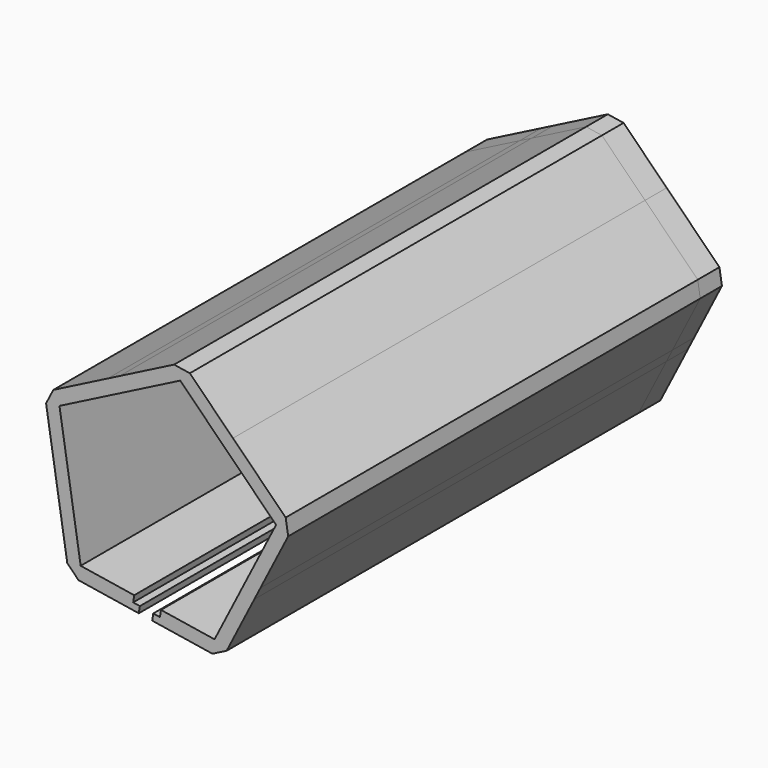
from build123d import *

# Parameters (mm, degrees)
F1_DEPTH = 101.6
F2_DEPTH = 5.08


with BuildPart() as f1:
    # F0 (on Front) → F1 (new body)
    with BuildSketch(Plane.XZ):
        Polygon((-28.6679874819, 40.9869131927), (-27.5148516125, 38.7237566213), (-4.8832858982, 50.2551153147), (-6.0364217675, 52.5182718861), (-16.220626339, 47.3291604741), (-18.4837829104, 46.1760246048), align=None)
        Polygon((-6.0364217675, 52.5182718861), (-4.8832858982, 50.2551153147), (-3.0872346739, 52.0511665389), align=None)
        Polygon((-3.0872346739, 52.0511665389), (-4.8832858982, 50.2551153147), (13.077226344, 32.2946030725), (14.8732775682, 34.0906542967), (6.7910470592, 42.1728848057), (4.994995835, 43.9689360299), align=None)
        Polygon((14.8732775682, 34.0906542967), (13.077226344, 32.2946030725), (15.3403829154, 31.1414672032), align=None)
        Polygon((15.3403829154, 31.1414672032), (13.077226344, 32.2946030725), (1.5458676506, 9.6630373581), (3.809024222, 8.5099014888), (8.9981356341, 18.6941060603), (10.1512715034, 20.9572626317), align=None)
        Polygon((-30.0235799977, 38.3264130801), (-27.5148516125, 38.7237566213), (-28.6679874819, 40.9869131927), align=None)
        Polygon((-23.5414162005, 13.6364727702), (-27.5148516125, 38.7237566213), (-30.0235799977, 38.3264130801), (-28.2355340622, 27.0371353471), (-27.838190521, 24.528406962), (-26.0501445856, 13.239129229), align=None)
        Polygon((-23.9387597417, 11.1277443851), (-23.5414162005, 13.6364727702), (-26.0501445856, 13.239129229), align=None)
        Polygon((-13.5065026601, 12.0470986054), (-23.5414162005, 13.6364727702), (-23.9387597417, 11.1277443851), (-12.6494820087, 9.3396984497), (-12.4508102381, 10.5940626422), (-13.7051744307, 10.7927344128), align=None)
        Polygon((3.809024222, 8.5099014888), (1.5458676506, 9.6630373581), (1.1485241094, 7.154308973), align=None)
        Polygon((1.5458676506, 9.6630373581), (-8.4890458899, 11.252411523), (-8.6877176605, 9.9980473304), (-9.942081853, 10.196719101), (-10.1407536236, 8.9423549084), (1.1485241094, 7.154308973), align=None)
    extrude(amount=F1_DEPTH)


with BuildPart() as f2:
    # F0 (on Front) → F2 (new body)
    with BuildSketch(Plane.XZ):
        Polygon((-4.8832858982, 50.2551153147), (-27.5148516125, 38.7237566213), (-23.5414162005, 13.6364727702), (-13.5065026601, 12.0470986054), (-8.4890458899, 11.252411523), (1.5458676506, 9.6630373581), (13.077226344, 32.2946030725), align=None)
        with BuildLine():
            add(Edge.make_bspline(
                [(-24.2410478902, 26.4475166861), (-24.1014147451, 26.5003988632), (-23.9344866256, 26.4169547892)],
                knots=[0, 0, 0, 1, 1, 1], degree=2))
            add(Edge.make_bspline(
                [(-23.9344866256, 26.4169547892), (-23.8245465392, 26.3619979088), (-23.763517385, 26.2778172496)],
                knots=[0, 0, 0, 1, 1, 1], degree=2))
            add(Edge.make_bspline(
                [(-23.763517385, 26.2778172496), (-23.7024882309, 26.1936365905), (-23.6979181512, 26.0929845147)],
                knots=[0, 0, 0, 1, 1, 1], degree=2))
            add(Edge.make_bspline(
                [(-23.6979181512, 26.0929845147), (-23.6933480715, 25.9923324389), (-23.7447541402, 25.8894956767)],
                knots=[0, 0, 0, 1, 1, 1], degree=2))
            Line((-23.7447541402, 25.8894956767), (-23.8776674766, 25.6236053355))
            Line((-23.8776674766, 25.6236053355), (-24.5884842175, 25.9789286021))
            Line((-24.5884842175, 25.9789286021), (-24.4709846317, 26.2139840586))
            add(Edge.make_bspline(
                [(-24.4709846317, 26.2139840586), (-24.3806810352, 26.394634509), (-24.2410478902, 26.4475166861)],
                knots=[0, 0, 0, 1, 1, 1], degree=2))
        make_face(mode=Mode.SUBTRACT)
        with BuildLine():
            Line((-23.5365275255, 26.9405958395), (-23.7311765646, 26.5512045201))
            add(Edge.make_bspline(
                [(-23.7311765646, 26.5512045201), (-23.6373803968, 26.5043176662), (-23.5669572, 26.517642507)],
                knots=[0, 0, 0, 1, 1, 1], degree=2))
            add(Edge.make_bspline(
                [(-23.5669572, 26.517642507), (-23.4965340031, 26.5309673477), (-23.4592504807, 26.6055522522)],
                knots=[0, 0, 0, 1, 1, 1], degree=2))
            add(Edge.make_bspline(
                [(-23.4592504807, 26.6055522522), (-23.4297141837, 26.6646389947), (-23.4356513358, 26.7120992744)],
                knots=[0, 0, 0, 1, 1, 1], degree=2))
            add(Edge.make_bspline(
                [(-23.4356513358, 26.7120992744), (-23.4415884879, 26.7595595541), (-23.4716176843, 26.7903093703)],
                knots=[0, 0, 0, 1, 1, 1], degree=2))
            Line((-23.4716176843, 26.7903093703), (-23.4092309675, 26.8586008524))
            add(Edge.make_bspline(
                [(-23.4092309675, 26.8586008524), (-23.3043703589, 26.7450438665), (-23.3911231438, 26.5714967404)],
                knots=[0, 0, 0, 1, 1, 1], degree=2))
            add(Edge.make_bspline(
                [(-23.3911231438, 26.5714967404), (-23.4516483425, 26.45041735), (-23.555446163, 26.4232062071)],
                knots=[0, 0, 0, 1, 1, 1], degree=2))
            add(Edge.make_bspline(
                [(-23.555446163, 26.4232062071), (-23.6592439835, 26.3959950642), (-23.8016333465, 26.4671726979)],
                knots=[0, 0, 0, 1, 1, 1], degree=2))
            add(Edge.make_bspline(
                [(-23.8016333465, 26.4671726979), (-23.9367579462, 26.5347188197), (-23.9772867589, 26.6340759995)],
                knots=[0, 0, 0, 1, 1, 1], degree=2))
            add(Edge.make_bspline(
                [(-23.9772867589, 26.6340759995), (-24.0178155717, 26.7334331793), (-23.9590657788, 26.8509609075)],
                knots=[0, 0, 0, 1, 1, 1], degree=2))
            add(Edge.make_bspline(
                [(-23.9590657788, 26.8509609075), (-23.8387416837, 27.0916667355), (-23.5486354645, 26.9466483593)],
                knots=[0, 0, 0, 1, 1, 1], degree=2))
            Line((-23.5486354645, 26.9466483593), (-23.5365275255, 26.9405958395))
        make_face(mode=Mode.SUBTRACT)
        with BuildLine():
            add(Edge.make_bspline(
                [(-23.2318323679, 27.4320627384), (-23.2023305644, 27.4299265975), (-23.1710113621, 27.4142707461)],
                knots=[0, 0, 0, 1, 1, 1], degree=2))
            add(Edge.make_bspline(
                [(-23.1710113621, 27.4142707461), (-23.0938434307, 27.3756960194), (-23.0810827573, 27.2964747541)],
                knots=[0, 0, 0, 1, 1, 1], degree=2))
            add(Edge.make_bspline(
                [(-23.0810827573, 27.2964747541), (-23.0683220839, 27.2172534888), (-23.1207772561, 27.1123180172)],
                knots=[0, 0, 0, 1, 1, 1], degree=2))
            add(Edge.make_bspline(
                [(-23.1207772561, 27.1123180172), (-23.1716991233, 27.0104498901), (-23.232918315, 26.9719426237)],
                knots=[0, 0, 0, 1, 1, 1], degree=2))
            add(Edge.make_bspline(
                [(-23.232918315, 26.9719426237), (-23.2941375067, 26.9334353572), (-23.3736443155, 26.9523959378)],
                knots=[0, 0, 0, 1, 1, 1], degree=2))
            Line((-23.3736443155, 26.9523959378), (-23.3491958849, 27.0404591395))
            add(Edge.make_bspline(
                [(-23.3491958849, 27.0404591395), (-23.299474007, 27.0301322889), (-23.2608943902, 27.0562475224)],
                knots=[0, 0, 0, 1, 1, 1], degree=2))
            add(Edge.make_bspline(
                [(-23.2608943902, 27.0562475224), (-23.2223147734, 27.082362756), (-23.1900346674, 27.1469384309)],
                knots=[0, 0, 0, 1, 1, 1], degree=2))
            add(Edge.make_bspline(
                [(-23.1900346674, 27.1469384309), (-23.155494954, 27.216034403), (-23.1606244849, 27.2586518163)],
                knots=[0, 0, 0, 1, 1, 1], degree=2))
            add(Edge.make_bspline(
                [(-23.1606244849, 27.2586518163), (-23.1657540158, 27.3012692297), (-23.208212522, 27.3224933994)],
                knots=[0, 0, 0, 1, 1, 1], degree=2))
            add(Edge.make_bspline(
                [(-23.208212522, 27.3224933994), (-23.2405003595, 27.3386334523), (-23.2717765443, 27.3265230972)],
                knots=[0, 0, 0, 1, 1, 1], degree=2))
            add(Edge.make_bspline(
                [(-23.2717765443, 27.3265230972), (-23.3030527291, 27.3144127421), (-23.3408235843, 27.2715490723)],
                knots=[0, 0, 0, 1, 1, 1], degree=2))
            Line((-23.3408235843, 27.2715490723), (-23.390458345, 27.215043308))
            add(Edge.make_bspline(
                [(-23.390458345, 27.215043308), (-23.4497778719, 27.1468328354), (-23.4857344981, 27.1235429035)],
                knots=[0, 0, 0, 1, 1, 1], degree=2))
            add(Edge.make_bspline(
                [(-23.4857344981, 27.1235429035), (-23.5216911243, 27.1002529717), (-23.5587795451, 27.0954871912)],
                knots=[0, 0, 0, 1, 1, 1], degree=2))
            add(Edge.make_bspline(
                [(-23.5587795451, 27.0954871912), (-23.5958679659, 27.0907214106), (-23.6362277627, 27.1108964769)],
                knots=[0, 0, 0, 1, 1, 1], degree=2))
            add(Edge.make_bspline(
                [(-23.6362277627, 27.1108964769), (-23.7108126671, 27.1481799993), (-23.7232902131, 27.2209036756)],
                knots=[0, 0, 0, 1, 1, 1], degree=2))
            add(Edge.make_bspline(
                [(-23.7232902131, 27.2209036756), (-23.7357677591, 27.2936273518), (-23.6848458919, 27.3954954789)],
                knots=[0, 0, 0, 1, 1, 1], degree=2))
            add(Edge.make_bspline(
                [(-23.6848458919, 27.3954954789), (-23.6396537435, 27.4859014237), (-23.5813402059, 27.5232380338)],
                knots=[0, 0, 0, 1, 1, 1], degree=2))
            add(Edge.make_bspline(
                [(-23.5813402059, 27.5232380338), (-23.5230266683, 27.5605746439), (-23.4457796989, 27.5395152379)],
                knots=[0, 0, 0, 1, 1, 1], degree=2))
            Line((-23.4457796989, 27.5395152379), (-23.4766048034, 27.4528235928))
            add(Edge.make_bspline(
                [(-23.4766048034, 27.4528235928), (-23.5167215329, 27.4633935106), (-23.5525974396, 27.4400632286)],
                knots=[0, 0, 0, 1, 1, 1], degree=2))
            add(Edge.make_bspline(
                [(-23.5525974396, 27.4400632286), (-23.5884733462, 27.4167329467), (-23.6162342374, 27.3611978663)],
                knots=[0, 0, 0, 1, 1, 1], degree=2))
            add(Edge.make_bspline(
                [(-23.6162342374, 27.3611978663), (-23.6469810383, 27.299689536), (-23.6429819103, 27.2610674429)],
                knots=[0, 0, 0, 1, 1, 1], degree=2))
            add(Edge.make_bspline(
                [(-23.6429819103, 27.2610674429), (-23.6389827823, 27.2224453499), (-23.6012060125, 27.2035614879)],
                knots=[0, 0, 0, 1, 1, 1], degree=2))
            add(Edge.make_bspline(
                [(-23.6012060125, 27.2035614879), (-23.5779587695, 27.1919406497), (-23.5568116857, 27.196503114)],
                knots=[0, 0, 0, 1, 1, 1], degree=2))
            add(Edge.make_bspline(
                [(-23.5568116857, 27.196503114), (-23.5356646018, 27.2010655782), (-23.5131466765, 27.2194709213)],
                knots=[0, 0, 0, 1, 1, 1], degree=2))
            add(Edge.make_bspline(
                [(-23.5131466765, 27.2194709213), (-23.4906287512, 27.2378762643), (-23.4339727196, 27.3047950301)],
                knots=[0, 0, 0, 1, 1, 1], degree=2))
            add(Edge.make_bspline(
                [(-23.4339727196, 27.3047950301), (-23.379657073, 27.3678392168), (-23.3484223981, 27.3919762115)],
                knots=[0, 0, 0, 1, 1, 1], degree=2))
            add(Edge.make_bspline(
                [(-23.3484223981, 27.3919762115), (-23.3171877231, 27.4161132062), (-23.2892609472, 27.4251560428)],
                knots=[0, 0, 0, 1, 1, 1], degree=2))
            add(Edge.make_bspline(
                [(-23.2892609472, 27.4251560428), (-23.2613341713, 27.4341988794), (-23.2318323679, 27.4320627384)],
                knots=[0, 0, 0, 1, 1, 1], degree=2))
        make_face(mode=Mode.SUBTRACT)
        Polygon((-22.9216114376, 27.5361753853), (-22.9670456868, 27.4452851229), (-23.5128715784, 27.7181327188), (-23.4674373292, 27.8090229811), align=None, mode=Mode.SUBTRACT)
        Polygon((-23.5835121048, 27.8670464716), (-23.6289463539, 27.7761562093), (-23.7158006366, 27.8195729518), (-23.6703663874, 27.9104632142), align=None, mode=Mode.SUBTRACT)
        with BuildLine():
            add(Edge.make_bspline(
                [(-22.6500587957, 28.1185653779), (-22.4200079541, 28.0035675003), (-22.534198829, 27.7751310506)],
                knots=[0, 0, 0, 1, 1, 1], degree=2))
            add(Edge.make_bspline(
                [(-22.534198829, 27.7751310506), (-22.5789067758, 27.6856937409), (-22.6404087663, 27.650253645)],
                knots=[0, 0, 0, 1, 1, 1], degree=2))
            add(Edge.make_bspline(
                [(-22.6404087663, 27.650253645), (-22.7019107568, 27.6148135492), (-22.7740722566, 27.6319183716)],
                knots=[0, 0, 0, 1, 1, 1], degree=2))
            Line((-22.7740722566, 27.6319183716), (-22.7414724808, 27.7298296729))
            add(Edge.make_bspline(
                [(-22.7414724808, 27.7298296729), (-22.6991764961, 27.7199864054), (-22.663219638, 27.7408548654)],
                knots=[0, 0, 0, 1, 1, 1], degree=2))
            add(Edge.make_bspline(
                [(-22.663219638, 27.7408548654), (-22.6272627798, 27.7617233254), (-22.6020842971, 27.8120923518)],
                knots=[0, 0, 0, 1, 1, 1], degree=2))
            add(Edge.make_bspline(
                [(-22.6020842971, 27.8120923518), (-22.5342153743, 27.9478627082), (-22.6930715344, 28.0272717689)],
                knots=[0, 0, 0, 1, 1, 1], degree=2))
            Line((-22.6930715344, 28.0272717689), (-22.7808944522, 28.071172713))
            Line((-22.7808944522, 28.071172713), (-22.7813786538, 28.0702040779))
            add(Edge.make_bspline(
                [(-22.7813786538, 28.0702040779), (-22.7418229604, 28.0181462218), (-22.7377816073, 27.9600312844)],
                knots=[0, 0, 0, 1, 1, 1], degree=2))
            add(Edge.make_bspline(
                [(-22.7377816073, 27.9600312844), (-22.7337402543, 27.9019163469), (-22.7637607529, 27.8418609693)],
                knots=[0, 0, 0, 1, 1, 1], degree=2))
            add(Edge.make_bspline(
                [(-22.7637607529, 27.8418609693), (-22.8139563177, 27.7414457949), (-22.9041144597, 27.7275944116)],
                knots=[0, 0, 0, 1, 1, 1], degree=2))
            add(Edge.make_bspline(
                [(-22.9041144597, 27.7275944116), (-22.9942726018, 27.7137430282), (-23.1369848432, 27.7850820625)],
                knots=[0, 0, 0, 1, 1, 1], degree=2))
            add(Edge.make_bspline(
                [(-23.1369848432, 27.7850820625), (-23.2817957941, 27.8574702001), (-23.3253097242, 27.9425807679)],
                knots=[0, 0, 0, 1, 1, 1], degree=2))
            add(Edge.make_bspline(
                [(-23.3253097242, 27.9425807679), (-23.3688236543, 28.0276913357), (-23.3170947844, 28.1311738546)],
                knots=[0, 0, 0, 1, 1, 1], degree=2))
            add(Edge.make_bspline(
                [(-23.3170947844, 28.1311738546), (-23.2881233893, 28.1891305228), (-23.2403424927, 28.2185156247)],
                knots=[0, 0, 0, 1, 1, 1], degree=2))
            add(Edge.make_bspline(
                [(-23.2403424927, 28.2185156247), (-23.192561596, 28.2479007267), (-23.1320246842, 28.2466957893)],
                knots=[0, 0, 0, 1, 1, 1], degree=2))
            Line((-23.1320246842, 28.2466957893), (-23.1315404826, 28.2476644244))
            add(Edge.make_bspline(
                [(-23.1315404826, 28.2476644244), (-23.1467157662, 28.2552502494), (-23.1829994651, 28.2759100004)],
                knots=[0, 0, 0, 1, 1, 1], degree=2))
            add(Edge.make_bspline(
                [(-23.1829994651, 28.2759100004), (-23.219283164, 28.2965697514), (-23.2217857227, 28.3004438667)],
                knots=[0, 0, 0, 1, 1, 1], degree=2))
            Line((-23.2217857227, 28.3004438667), (-23.1786917812, 28.3866523926))
            add(Edge.make_bspline(
                [(-23.1786917812, 28.3866523926), (-23.1531033028, 28.3700274036), (-23.0672176552, 28.3270948626)],
                knots=[0, 0, 0, 1, 1, 1], degree=2))
            Line((-23.0672176552, 28.3270948626), (-22.6500587957, 28.1185653779))
        make_face(mode=Mode.SUBTRACT)
        with BuildLine():
            Line((-22.3458957473, 28.6878825462), (-22.3915720973, 28.5965079663))
            Line((-22.3915720973, 28.5965079663), (-22.7376977145, 28.7695293343))
            add(Edge.make_bspline(
                [(-22.7376977145, 28.7695293343), (-22.791618403, 28.7964832228), (-22.8266898003, 28.800798155)],
                knots=[0, 0, 0, 1, 1, 1], degree=2))
            add(Edge.make_bspline(
                [(-22.8266898003, 28.800798155), (-22.8617611977, 28.8051130871), (-22.88645861, 28.7884025656)],
                knots=[0, 0, 0, 1, 1, 1], degree=2))
            add(Edge.make_bspline(
                [(-22.88645861, 28.7884025656), (-22.9111560223, 28.7716920441), (-22.933590696, 28.7268119501)],
                knots=[0, 0, 0, 1, 1, 1], degree=2))
            add(Edge.make_bspline(
                [(-22.933590696, 28.7268119501), (-22.9663550036, 28.6612676402), (-22.9403991217, 28.6009754771)],
                knots=[0, 0, 0, 1, 1, 1], degree=2))
            add(Edge.make_bspline(
                [(-22.9403991217, 28.6009754771), (-22.9144432398, 28.5406833141), (-22.8346922814, 28.5008173832)],
                knots=[0, 0, 0, 1, 1, 1], degree=2))
            Line((-22.8346922814, 28.5008173832), (-22.5184329138, 28.3427255641))
            Line((-22.5184329138, 28.3427255641), (-22.5637864627, 28.251996741))
            Line((-22.5637864627, 28.251996741), (-22.9930532613, 28.4665787455))
            add(Edge.make_bspline(
                [(-22.9930532613, 28.4665787455), (-23.0884638209, 28.5142726021), (-23.1111456594, 28.5217769922)],
                knots=[0, 0, 0, 1, 1, 1], degree=2))
            Line((-23.1111456594, 28.5217769922), (-23.0682938187, 28.6075012006))
            add(Edge.make_bspline(
                [(-23.0682938187, 28.6075012006), (-23.0656301301, 28.6067750142), (-23.0542083753, 28.6017717331)],
                knots=[0, 0, 0, 1, 1, 1], degree=2))
            add(Edge.make_bspline(
                [(-23.0542083753, 28.6017717331), (-23.0427866204, 28.5967684519), (-23.0280553816, 28.5903126047)],
                knots=[0, 0, 0, 1, 1, 1], degree=2))
            add(Edge.make_bspline(
                [(-23.0280553816, 28.5903126047), (-23.0133241427, 28.5838567575), (-22.9729644619, 28.5648924271)],
                knots=[0, 0, 0, 1, 1, 1], degree=2))
            Line((-22.9729644619, 28.5648924271), (-22.9721574593, 28.566506819))
            add(Edge.make_bspline(
                [(-22.9721574593, 28.566506819), (-23.0130860236, 28.6259096749), (-23.0159968578, 28.6788185561)],
                knots=[0, 0, 0, 1, 1, 1], degree=2))
            add(Edge.make_bspline(
                [(-23.0159968578, 28.6788185561), (-23.0189076919, 28.7317274374), (-22.9884029918, 28.7927514501)],
                knots=[0, 0, 0, 1, 1, 1], degree=2))
            add(Edge.make_bspline(
                [(-22.9884029918, 28.7927514501), (-22.9435336445, 28.8825116382), (-22.8780750409, 28.9018493252)],
                knots=[0, 0, 0, 1, 1, 1], degree=2))
            add(Edge.make_bspline(
                [(-22.8780750409, 28.9018493252), (-22.8126164373, 28.9211870122), (-22.7096182359, 28.8697002431)],
                knots=[0, 0, 0, 1, 1, 1], degree=2))
            Line((-22.7096182359, 28.8697002431), (-22.3458957473, 28.6878825462))
        make_face(mode=Mode.SUBTRACT)
        with BuildLine():
            Line((-22.3018941717, 29.4104539632), (-22.4965432108, 29.0210626438))
            add(Edge.make_bspline(
                [(-22.4965432108, 29.0210626438), (-22.4027470431, 28.9741757899), (-22.3323238463, 28.9875006307)],
                knots=[0, 0, 0, 1, 1, 1], degree=2))
            add(Edge.make_bspline(
                [(-22.3323238463, 28.9875006307), (-22.2619006494, 29.0008254714), (-22.224617127, 29.0754103759)],
                knots=[0, 0, 0, 1, 1, 1], degree=2))
            add(Edge.make_bspline(
                [(-22.224617127, 29.0754103759), (-22.19508083, 29.1344971184), (-22.2010179821, 29.1819573981)],
                knots=[0, 0, 0, 1, 1, 1], degree=2))
            add(Edge.make_bspline(
                [(-22.2010179821, 29.1819573981), (-22.2069551342, 29.2294176778), (-22.2369843306, 29.260167494)],
                knots=[0, 0, 0, 1, 1, 1], degree=2))
            Line((-22.2369843306, 29.260167494), (-22.1745976138, 29.3284589761))
            add(Edge.make_bspline(
                [(-22.1745976138, 29.3284589761), (-22.0697370052, 29.2149019902), (-22.15648979, 29.0413548641)],
                knots=[0, 0, 0, 1, 1, 1], degree=2))
            add(Edge.make_bspline(
                [(-22.15648979, 29.0413548641), (-22.2170149888, 28.9202754737), (-22.3208128093, 28.8930643308)],
                knots=[0, 0, 0, 1, 1, 1], degree=2))
            add(Edge.make_bspline(
                [(-22.3208128093, 28.8930643308), (-22.4246106298, 28.8658531879), (-22.5669999928, 28.9370308216)],
                knots=[0, 0, 0, 1, 1, 1], degree=2))
            add(Edge.make_bspline(
                [(-22.5669999928, 28.9370308216), (-22.7021245924, 29.0045769434), (-22.7426534052, 29.1039341232)],
                knots=[0, 0, 0, 1, 1, 1], degree=2))
            add(Edge.make_bspline(
                [(-22.7426534052, 29.1039341232), (-22.783182218, 29.203291303), (-22.7244324251, 29.3208190312)],
                knots=[0, 0, 0, 1, 1, 1], degree=2))
            add(Edge.make_bspline(
                [(-22.7244324251, 29.3208190312), (-22.60410833, 29.5615248592), (-22.3140021108, 29.416506483)],
                knots=[0, 0, 0, 1, 1, 1], degree=2))
            Line((-22.3140021108, 29.416506483), (-22.3018941717, 29.4104539632))
        make_face(mode=Mode.SUBTRACT)
        with BuildLine():
            Line((-21.9049705291, 29.7895330443), (-21.9059389322, 29.7875957741))
            add(Edge.make_bspline(
                [(-21.9059389322, 29.7875957741), (-21.866141138, 29.7360222356), (-21.8641585309, 29.6830729075)],
                knots=[0, 0, 0, 1, 1, 1], degree=2))
            add(Edge.make_bspline(
                [(-21.8641585309, 29.6830729075), (-21.8621759237, 29.6301235795), (-21.8929227247, 29.5686152492)],
                knots=[0, 0, 0, 1, 1, 1], degree=2))
            add(Edge.make_bspline(
                [(-21.8929227247, 29.5686152492), (-21.9446515945, 29.4651327302), (-22.0386437336, 29.4512809797)],
                knots=[0, 0, 0, 1, 1, 1], degree=2))
            add(Edge.make_bspline(
                [(-22.0386437336, 29.4512809797), (-22.1326358728, 29.4374292291), (-22.2738951615, 29.5080419609)],
                knots=[0, 0, 0, 1, 1, 1], degree=2))
            add(Edge.make_bspline(
                [(-22.2738951615, 29.5080419609), (-22.5594810835, 29.6508007296), (-22.4590899539, 29.8516310784)],
                knots=[0, 0, 0, 1, 1, 1], degree=2))
            add(Edge.make_bspline(
                [(-22.4590899539, 29.8516310784), (-22.4281010521, 29.9136237263), (-22.3847595785, 29.9436137709)],
                knots=[0, 0, 0, 1, 1, 1], degree=2))
            add(Edge.make_bspline(
                [(-22.3847595785, 29.9436137709), (-22.3414181049, 29.9736038156), (-22.2791863328, 29.9741747867)],
                knots=[0, 0, 0, 1, 1, 1], degree=2))
            Line((-22.2791863328, 29.9741747867), (-22.2787021313, 29.9751434218))
            Line((-22.2787021313, 29.9751434218), (-22.3402103456, 30.0046794868))
            Line((-22.3402103456, 30.0046794868), (-22.5668709643, 30.1179826588))
            Line((-22.5668709643, 30.1179826588), (-22.5215174154, 30.208711482))
            Line((-22.5215174154, 30.208711482), (-21.8852855789, 29.8906717378))
            add(Edge.make_bspline(
                [(-21.8852855789, 29.8906717378), (-21.8000456882, 29.8480619979), (-21.7712291605, 29.8374909976)],
                knots=[0, 0, 0, 1, 1, 1], degree=2))
            Line((-21.7712291605, 29.8374909976), (-21.814645903, 29.750636715))
            add(Edge.make_bspline(
                [(-21.814645903, 29.750636715), (-21.8234441648, 29.7532187755), (-21.8536330802, 29.7660900426)],
                knots=[0, 0, 0, 1, 1, 1], degree=2))
            add(Edge.make_bspline(
                [(-21.8536330802, 29.7660900426), (-21.8838219955, 29.7789613096), (-21.9049705291, 29.7895330443)],
                knots=[0, 0, 0, 1, 1, 1], degree=2))
        make_face(mode=Mode.SUBTRACT)
        with BuildLine():
            add(Edge.make_bspline(
                [(-21.8395776893, 30.9167748155), (-21.7455855502, 30.9306265661), (-21.6043262614, 30.8600138342)],
                knots=[0, 0, 0, 1, 1, 1], degree=2))
            add(Edge.make_bspline(
                [(-21.6043262614, 30.8600138342), (-21.3187403394, 30.7172550655), (-21.419131469, 30.5164247168)],
                knots=[0, 0, 0, 1, 1, 1], degree=2))
            add(Edge.make_bspline(
                [(-21.419131469, 30.5164247168), (-21.4501203708, 30.4544320689), (-21.493219705, 30.4245227631)],
                knots=[0, 0, 0, 1, 1, 1], degree=2))
            add(Edge.make_bspline(
                [(-21.493219705, 30.4245227631), (-21.5363190391, 30.3946134574), (-21.5990350901, 30.3938810085)],
                knots=[0, 0, 0, 1, 1, 1], degree=2))
            Line((-21.5990350901, 30.3938810085), (-21.5995192917, 30.3929123734))
            add(Edge.make_bspline(
                [(-21.5995192917, 30.3929123734), (-21.5838596905, 30.3850844477), (-21.5528227652, 30.3670474553)],
                knots=[0, 0, 0, 1, 1, 1], degree=2))
            add(Edge.make_bspline(
                [(-21.5528227652, 30.3670474553), (-21.5217858399, 30.3490104628), (-21.5173461269, 30.3453786803)],
                knots=[0, 0, 0, 1, 1, 1], degree=2))
            Line((-21.5173461269, 30.3453786803), (-21.5611663708, 30.2577172017))
            add(Edge.make_bspline(
                [(-21.5611663708, 30.2577172017), (-21.5869969886, 30.2742614518), (-21.6722368794, 30.3168711917)],
                knots=[0, 0, 0, 1, 1, 1], degree=2))
            Line((-21.6722368794, 30.3168711917), (-22.3084687159, 30.634910936))
            Line((-22.3084687159, 30.634910936), (-22.2630344667, 30.7258011983))
            Line((-22.2630344667, 30.7258011983), (-22.0496118613, 30.619115448))
            add(Edge.make_bspline(
                [(-22.0496118613, 30.619115448), (-22.0168397063, 30.6027332942), (-21.9734930333, 30.578442012)],
                knots=[0, 0, 0, 1, 1, 1], degree=2))
            Line((-21.9734930333, 30.578442012), (-21.9724439299, 30.5805407214))
            add(Edge.make_bspline(
                [(-21.9724439299, 30.5805407214), (-22.0123224244, 30.6319528207), (-22.0141839618, 30.6849425182)],
                knots=[0, 0, 0, 1, 1, 1], degree=2))
            add(Edge.make_bspline(
                [(-22.0141839618, 30.6849425182), (-22.0160454992, 30.7379322157), (-21.9852986983, 30.799440546)],
                knots=[0, 0, 0, 1, 1, 1], degree=2))
            add(Edge.make_bspline(
                [(-21.9852986983, 30.799440546), (-21.9335698284, 30.9029230649), (-21.8395776893, 30.9167748155)],
                knots=[0, 0, 0, 1, 1, 1], degree=2))
        make_face(mode=Mode.SUBTRACT)
        with BuildLine():
            add(Edge.make_bspline(
                [(-21.0253913312, 30.8457422463), (-21.0222793649, 30.7996942212), (-21.0447140385, 30.7548141272)],
                knots=[0, 0, 0, 1, 1, 1], degree=2))
            add(Edge.make_bspline(
                [(-21.0447140385, 30.7548141272), (-21.0633557997, 30.717521675), (-21.0815146737, 30.6949195316)],
                knots=[0, 0, 0, 1, 1, 1], degree=2))
            Line((-21.0815146737, 30.6949195316), (-21.1496420107, 30.7289750434))
            add(Edge.make_bspline(
                [(-21.1496420107, 30.7289750434), (-21.1369713346, 30.7466530017), (-21.1253504964, 30.7699002446)],
                knots=[0, 0, 0, 1, 1, 1], degree=2))
            add(Edge.make_bspline(
                [(-21.1253504964, 30.7699002446), (-21.0829828573, 30.8546558178), (-21.1829196287, 30.9663568136)],
                knots=[0, 0, 0, 1, 1, 1], degree=2))
            Line((-21.1829196287, 30.9663568136), (-21.2004368049, 30.9858076263))
            Line((-21.2004368049, 30.9858076263), (-21.8518180246, 31.0410355072))
            Line((-21.8518180246, 31.0410355072), (-21.8033978656, 31.1378990195))
            Line((-21.8033978656, 31.1378990195), (-21.4443708754, 31.1020956257))
            add(Edge.make_bspline(
                [(-21.4443708754, 31.1020956257), (-21.435976347, 31.1011278411), (-21.4243531507, 31.099756787)],
                knots=[0, 0, 0, 1, 1, 1], degree=2))
            add(Edge.make_bspline(
                [(-21.4243531507, 31.099756787), (-21.4127299545, 31.098385733), (-21.3471475751, 31.0895132847)],
                knots=[0, 0, 0, 1, 1, 1], degree=2))
            add(Edge.make_bspline(
                [(-21.3471475751, 31.0895132847), (-21.2815651958, 31.0806408365), (-21.274381326, 31.0788657785)],
                knots=[0, 0, 0, 1, 1, 1], degree=2))
            Line((-21.274381326, 31.0788657785), (-21.355993068, 31.1638516235))
            Line((-21.355993068, 31.1638516235), (-21.6437727415, 31.4572257316))
            Line((-21.6437727415, 31.4572257316), (-21.5958367841, 31.5531206087))
            Line((-21.5958367841, 31.5531206087), (-21.1549212369, 31.0704020696))
            add(Edge.make_bspline(
                [(-21.1549212369, 31.0704020696), (-21.0845296924, 30.992840997), (-21.0565164949, 30.9423156342)],
                knots=[0, 0, 0, 1, 1, 1], degree=2))
            add(Edge.make_bspline(
                [(-21.0565164949, 30.9423156342), (-21.0285032975, 30.8917902714), (-21.0253913312, 30.8457422463)],
                knots=[0, 0, 0, 1, 1, 1], degree=2))
        make_face(mode=Mode.SUBTRACT)
        with BuildLine():
            add(Edge.make_bspline(
                [(-20.7628104206, 31.9777247755), (-20.7314845113, 31.8920480302), (-20.780146771, 31.7947002003)],
                knots=[0, 0, 0, 1, 1, 1], degree=2))
            add(Edge.make_bspline(
                [(-20.780146771, 31.7947002003), (-20.8704503675, 31.61404975), (-21.0741018624, 31.6736791664)],
                knots=[0, 0, 0, 1, 1, 1], degree=2))
            Line((-21.0741018624, 31.6736791664), (-21.0426325088, 31.7757875774))
            add(Edge.make_bspline(
                [(-21.0426325088, 31.7757875774), (-20.9794301688, 31.7556954149), (-20.9308004117, 31.7710360614)],
                knots=[0, 0, 0, 1, 1, 1], degree=2))
            add(Edge.make_bspline(
                [(-20.9308004117, 31.7710360614), (-20.8821706547, 31.7863767078), (-20.858202676, 31.8343241464)],
                knots=[0, 0, 0, 1, 1, 1], degree=2))
            add(Edge.make_bspline(
                [(-20.858202676, 31.8343241464), (-20.8319750899, 31.8867918822), (-20.8529254485, 31.935098239)],
                knots=[0, 0, 0, 1, 1, 1], degree=2))
            add(Edge.make_bspline(
                [(-20.8529254485, 31.935098239), (-20.8738758072, 31.9834045958), (-20.9434560968, 32.01818641)],
                knots=[0, 0, 0, 1, 1, 1], degree=2))
            Line((-20.9434560968, 32.01818641), (-21.3657810103, 32.2292983032))
            Line((-21.3657810103, 32.2292983032), (-21.4341341347, 32.0925593117))
            Line((-21.4341341347, 32.0925593117), (-21.5127550189, 32.1318603407))
            Line((-21.5127550189, 32.1318603407), (-21.396465937, 32.3644942094))
            Line((-21.396465937, 32.3644942094), (-20.8976188489, 32.1151303906))
            add(Edge.make_bspline(
                [(-20.8976188489, 32.1151303906), (-20.7941363299, 32.0634015208), (-20.7628104206, 31.9777247755)],
                knots=[0, 0, 0, 1, 1, 1], degree=2))
        make_face(mode=Mode.SUBTRACT)
        with BuildLine():
            Line((-20.6368056047, 32.7414287109), (-20.8314546438, 32.3520373916))
            add(Edge.make_bspline(
                [(-20.8314546438, 32.3520373916), (-20.7376584761, 32.3051505377), (-20.6672352792, 32.3184753784)],
                knots=[0, 0, 0, 1, 1, 1], degree=2))
            add(Edge.make_bspline(
                [(-20.6672352792, 32.3184753784), (-20.5968120824, 32.3318002192), (-20.55952856, 32.4063851237)],
                knots=[0, 0, 0, 1, 1, 1], degree=2))
            add(Edge.make_bspline(
                [(-20.55952856, 32.4063851237), (-20.529992263, 32.4654718661), (-20.5359294151, 32.5129321459)],
                knots=[0, 0, 0, 1, 1, 1], degree=2))
            add(Edge.make_bspline(
                [(-20.5359294151, 32.5129321459), (-20.5418665671, 32.5603924256), (-20.5718957636, 32.5911422418)],
                knots=[0, 0, 0, 1, 1, 1], degree=2))
            Line((-20.5718957636, 32.5911422418), (-20.5095090467, 32.6594337239))
            add(Edge.make_bspline(
                [(-20.5095090467, 32.6594337239), (-20.4046484382, 32.545876738), (-20.491401223, 32.3723296118)],
                knots=[0, 0, 0, 1, 1, 1], degree=2))
            add(Edge.make_bspline(
                [(-20.491401223, 32.3723296118), (-20.5519264217, 32.2512502215), (-20.6557242422, 32.2240390786)],
                knots=[0, 0, 0, 1, 1, 1], degree=2))
            add(Edge.make_bspline(
                [(-20.6557242422, 32.2240390786), (-20.7595220627, 32.1968279357), (-20.9019114258, 32.2680055694)],
                knots=[0, 0, 0, 1, 1, 1], degree=2))
            add(Edge.make_bspline(
                [(-20.9019114258, 32.2680055694), (-21.0370360254, 32.3355516912), (-21.0775648382, 32.434908871)],
                knots=[0, 0, 0, 1, 1, 1], degree=2))
            add(Edge.make_bspline(
                [(-21.0775648382, 32.434908871), (-21.1180936509, 32.5342660507), (-21.059343858, 32.651793779)],
                knots=[0, 0, 0, 1, 1, 1], degree=2))
            add(Edge.make_bspline(
                [(-21.059343858, 32.651793779), (-20.939019763, 32.892499607), (-20.6489135437, 32.7474812308)],
                knots=[0, 0, 0, 1, 1, 1], degree=2))
            Line((-20.6489135437, 32.7474812308), (-20.6368056047, 32.7414287109))
        make_face(mode=Mode.SUBTRACT)
        with BuildLine():
            Line((-20.6956095176, 33.1889110776), (-20.7488716925, 33.0823612141))
            Line((-20.7488716925, 33.0823612141), (-20.2690744284, 32.8425200266))
            Line((-20.2690744284, 32.8425200266), (-20.3144279773, 32.7517912035))
            Line((-20.3144279773, 32.7517912035), (-20.7942252414, 32.9916323909))
            Line((-20.7942252414, 32.9916323909), (-20.8325578673, 32.9149487771))
            Line((-20.8325578673, 32.9149487771), (-20.8985864948, 32.9479551854))
            Line((-20.8985864948, 32.9479551854), (-20.860253869, 33.0246387993))
            Line((-20.860253869, 33.0246387993), (-20.9219236384, 33.0554663005))
            add(Edge.make_bspline(
                [(-20.9219236384, 33.0554663005), (-20.9965085429, 33.0927498229), (-21.0128985441, 33.1419041317)],
                knots=[0, 0, 0, 1, 1, 1], degree=2))
            add(Edge.make_bspline(
                [(-21.0128985441, 33.1419041317), (-21.0292885453, 33.1910584405), (-20.9954751343, 33.2587014599)],
                knots=[0, 0, 0, 1, 1, 1], degree=2))
            add(Edge.make_bspline(
                [(-20.9954751343, 33.2587014599), (-20.9765912723, 33.2964782297), (-20.9574638791, 33.3198069074)],
                knots=[0, 0, 0, 1, 1, 1], degree=2))
            Line((-20.9574638791, 33.3198069074), (-20.8883679071, 33.285267194))
            add(Edge.make_bspline(
                [(-20.8883679071, 33.285267194), (-20.9037826241, 33.2645217752), (-20.912578953, 33.2469249038)],
                knots=[0, 0, 0, 1, 1, 1], degree=2))
            add(Edge.make_bspline(
                [(-20.912578953, 33.2469249038), (-20.9300102102, 33.2120540394), (-20.9201605449, 33.1875577592)],
                knots=[0, 0, 0, 1, 1, 1], degree=2))
            add(Edge.make_bspline(
                [(-20.9201605449, 33.1875577592), (-20.9103108796, 33.1630614791), (-20.8638163938, 33.1398198028)],
                knots=[0, 0, 0, 1, 1, 1], degree=2))
            Line((-20.8638163938, 33.1398198028), (-20.8149003201, 33.1153676225))
            Line((-20.8149003201, 33.1153676225), (-20.7616381452, 33.221917486))
            Line((-20.7616381452, 33.221917486), (-20.6956095176, 33.1889110776))
        make_face(mode=Mode.SUBTRACT)
        with BuildLine():
            Line((-20.5521244465, 33.4759499523), (-20.6053866214, 33.3694000888))
            Line((-20.6053866214, 33.3694000888), (-20.1255893573, 33.1295589013))
            Line((-20.1255893573, 33.1295589013), (-20.1709429062, 33.0388300782))
            Line((-20.1709429062, 33.0388300782), (-20.6507401703, 33.2786712656))
            Line((-20.6507401703, 33.2786712656), (-20.6890727962, 33.2019876518))
            Line((-20.6890727962, 33.2019876518), (-20.7551014237, 33.2349940601))
            Line((-20.7551014237, 33.2349940601), (-20.7167687979, 33.311677674))
            Line((-20.7167687979, 33.311677674), (-20.7784385673, 33.3425051752))
            add(Edge.make_bspline(
                [(-20.7784385673, 33.3425051752), (-20.8530234718, 33.3797886976), (-20.869413473, 33.4289430064)],
                knots=[0, 0, 0, 1, 1, 1], degree=2))
            add(Edge.make_bspline(
                [(-20.869413473, 33.4289430064), (-20.8858034742, 33.4780973152), (-20.8519900632, 33.5457403346)],
                knots=[0, 0, 0, 1, 1, 1], degree=2))
            add(Edge.make_bspline(
                [(-20.8519900632, 33.5457403346), (-20.8331062012, 33.5835171044), (-20.813978808, 33.6068457821)],
                knots=[0, 0, 0, 1, 1, 1], degree=2))
            Line((-20.813978808, 33.6068457821), (-20.744882836, 33.5723060687))
            add(Edge.make_bspline(
                [(-20.744882836, 33.5723060687), (-20.760297553, 33.5515606499), (-20.7690938819, 33.5339637785)],
                knots=[0, 0, 0, 1, 1, 1], degree=2))
            add(Edge.make_bspline(
                [(-20.7690938819, 33.5339637785), (-20.7865251391, 33.4990929141), (-20.7766754738, 33.4745966339)],
                knots=[0, 0, 0, 1, 1, 1], degree=2))
            add(Edge.make_bspline(
                [(-20.7766754738, 33.4745966339), (-20.7668258085, 33.4501003538), (-20.7203313226, 33.4268586775)],
                knots=[0, 0, 0, 1, 1, 1], degree=2))
            Line((-20.7203313226, 33.4268586775), (-20.6714152489, 33.4024064972))
            Line((-20.6714152489, 33.4024064972), (-20.6181530741, 33.5089563607))
            Line((-20.6181530741, 33.5089563607), (-20.5521244465, 33.4759499523))
        make_face(mode=Mode.SUBTRACT)
        with BuildLine():
            Line((-20.0626232195, 33.8900685273), (-20.2572722586, 33.500677208))
            add(Edge.make_bspline(
                [(-20.2572722586, 33.500677208), (-20.1634760908, 33.453790354), (-20.093052894, 33.4671151948)],
                knots=[0, 0, 0, 1, 1, 1], degree=2))
            add(Edge.make_bspline(
                [(-20.093052894, 33.4671151948), (-20.0226296971, 33.4804400356), (-19.9853461747, 33.55502494)],
                knots=[0, 0, 0, 1, 1, 1], degree=2))
            add(Edge.make_bspline(
                [(-19.9853461747, 33.55502494), (-19.9558098777, 33.6141116825), (-19.9617470298, 33.6615719622)],
                knots=[0, 0, 0, 1, 1, 1], degree=2))
            add(Edge.make_bspline(
                [(-19.9617470298, 33.6615719622), (-19.9676841819, 33.7090322419), (-19.9977133783, 33.7397820581)],
                knots=[0, 0, 0, 1, 1, 1], degree=2))
            Line((-19.9977133783, 33.7397820581), (-19.9353266615, 33.8080735403))
            add(Edge.make_bspline(
                [(-19.9353266615, 33.8080735403), (-19.8304660529, 33.6945165543), (-19.9172188378, 33.5209694282)],
                knots=[0, 0, 0, 1, 1, 1], degree=2))
            add(Edge.make_bspline(
                [(-19.9172188378, 33.5209694282), (-19.9777440365, 33.3998900378), (-20.081541857, 33.3726788949)],
                knots=[0, 0, 0, 1, 1, 1], degree=2))
            add(Edge.make_bspline(
                [(-20.081541857, 33.3726788949), (-20.1853396775, 33.345467752), (-20.3277290405, 33.4166453857)],
                knots=[0, 0, 0, 1, 1, 1], degree=2))
            add(Edge.make_bspline(
                [(-20.3277290405, 33.4166453857), (-20.4628536402, 33.4841915075), (-20.5033824529, 33.5835486873)],
                knots=[0, 0, 0, 1, 1, 1], degree=2))
            add(Edge.make_bspline(
                [(-20.5033824529, 33.5835486873), (-20.5439112657, 33.6829058671), (-20.4851614728, 33.8004335953)],
                knots=[0, 0, 0, 1, 1, 1], degree=2))
            add(Edge.make_bspline(
                [(-20.4851614728, 33.8004335953), (-20.3648373777, 34.0411394233), (-20.0747311585, 33.8961210472)],
                knots=[0, 0, 0, 1, 1, 1], degree=2))
            Line((-20.0747311585, 33.8961210472), (-20.0626232195, 33.8900685273))
        make_face(mode=Mode.SUBTRACT)
        with BuildLine():
            Line((-19.7047374755, 33.9714642621), (-19.7500910244, 33.880735439))
            Line((-19.7500910244, 33.880735439), (-20.1688642758, 34.0900719263))
            add(Edge.make_bspline(
                [(-20.1688642758, 34.0900719263), (-20.2263366264, 34.1188012206), (-20.2974502211, 34.1505156903)],
                knots=[0, 0, 0, 1, 1, 1], degree=2))
            Line((-20.2974502211, 34.1505156903), (-20.2545983804, 34.2362398986))
            add(Edge.make_bspline(
                [(-20.2545983804, 34.2362398986), (-20.1597533412, 34.193873226), (-20.1411878347, 34.1845926955)],
                knots=[0, 0, 0, 1, 1, 1], degree=2))
            Line((-20.1411878347, 34.1845926955), (-20.1401387312, 34.1866914049))
            add(Edge.make_bspline(
                [(-20.1401387312, 34.1866914049), (-20.1993895029, 34.243348171), (-20.2110165069, 34.284471721)],
                knots=[0, 0, 0, 1, 1, 1], degree=2))
            add(Edge.make_bspline(
                [(-20.2110165069, 34.284471721), (-20.2226435109, 34.325595271), (-20.1969001263, 34.3770943717)],
                knots=[0, 0, 0, 1, 1, 1], degree=2))
            add(Edge.make_bspline(
                [(-20.1969001263, 34.3770943717), (-20.1878616967, 34.3951755606), (-20.1734958511, 34.4114007981)],
                knots=[0, 0, 0, 1, 1, 1], degree=2))
            Line((-20.1734958511, 34.4114007981), (-20.0901932306, 34.3697594614))
            add(Edge.make_bspline(
                [(-20.0901932306, 34.3697594614), (-20.1042362751, 34.3541799807), (-20.1194079249, 34.3238294135)],
                knots=[0, 0, 0, 1, 1, 1], degree=2))
            add(Edge.make_bspline(
                [(-20.1194079249, 34.3238294135), (-20.1476530176, 34.267325698), (-20.1138683016, 34.2132090381)],
                knots=[0, 0, 0, 1, 1, 1], degree=2))
            add(Edge.make_bspline(
                [(-20.1138683016, 34.2132090381), (-20.0800835856, 34.1590923782), (-19.9893547624, 34.1137388293)],
                knots=[0, 0, 0, 1, 1, 1], degree=2))
            Line((-19.9893547624, 34.1137388293), (-19.7047374755, 33.9714642621))
        make_face(mode=Mode.SUBTRACT)
        with BuildLine():
            add(Edge.make_bspline(
                [(-19.5859557972, 34.725562334), (-19.5564539938, 34.7234261931), (-19.5251347915, 34.7077703417)],
                knots=[0, 0, 0, 1, 1, 1], degree=2))
            add(Edge.make_bspline(
                [(-19.5251347915, 34.7077703417), (-19.4479668601, 34.669195615), (-19.4352061867, 34.5899743497)],
                knots=[0, 0, 0, 1, 1, 1], degree=2))
            add(Edge.make_bspline(
                [(-19.4352061867, 34.5899743497), (-19.4224455132, 34.5107530844), (-19.4749006855, 34.4058176128)],
                knots=[0, 0, 0, 1, 1, 1], degree=2))
            add(Edge.make_bspline(
                [(-19.4749006855, 34.4058176128), (-19.5258225527, 34.3039494857), (-19.5870417443, 34.2654422192)],
                knots=[0, 0, 0, 1, 1, 1], degree=2))
            add(Edge.make_bspline(
                [(-19.5870417443, 34.2654422192), (-19.648260936, 34.2269349528), (-19.7277677448, 34.2458955333)],
                knots=[0, 0, 0, 1, 1, 1], degree=2))
            Line((-19.7277677448, 34.2458955333), (-19.7033193143, 34.333958735))
            add(Edge.make_bspline(
                [(-19.7033193143, 34.333958735), (-19.6535974363, 34.3236318844), (-19.6150178195, 34.349747118)],
                knots=[0, 0, 0, 1, 1, 1], degree=2))
            add(Edge.make_bspline(
                [(-19.6150178195, 34.349747118), (-19.5764382027, 34.3758623516), (-19.5441580967, 34.4404380264)],
                knots=[0, 0, 0, 1, 1, 1], degree=2))
            add(Edge.make_bspline(
                [(-19.5441580967, 34.4404380264), (-19.5096183833, 34.5095339985), (-19.5147479143, 34.5521514119)],
                knots=[0, 0, 0, 1, 1, 1], degree=2))
            add(Edge.make_bspline(
                [(-19.5147479143, 34.5521514119), (-19.5198774452, 34.5947688252), (-19.5623359514, 34.6159929949)],
                knots=[0, 0, 0, 1, 1, 1], degree=2))
            add(Edge.make_bspline(
                [(-19.5623359514, 34.6159929949), (-19.5946237888, 34.6321330479), (-19.6258999736, 34.6200226928)],
                knots=[0, 0, 0, 1, 1, 1], degree=2))
            add(Edge.make_bspline(
                [(-19.6258999736, 34.6200226928), (-19.6571761585, 34.6079123377), (-19.6949470137, 34.5650486679)],
                knots=[0, 0, 0, 1, 1, 1], degree=2))
            Line((-19.6949470137, 34.5650486679), (-19.7445817743, 34.5085429036))
            add(Edge.make_bspline(
                [(-19.7445817743, 34.5085429036), (-19.8039013012, 34.440332431), (-19.8398579274, 34.4170424991)],
                knots=[0, 0, 0, 1, 1, 1], degree=2))
            add(Edge.make_bspline(
                [(-19.8398579274, 34.4170424991), (-19.8758145537, 34.3937525673), (-19.9129029745, 34.3889867867)],
                knots=[0, 0, 0, 1, 1, 1], degree=2))
            add(Edge.make_bspline(
                [(-19.9129029745, 34.3889867867), (-19.9499913952, 34.3842210062), (-19.990351192, 34.4043960724)],
                knots=[0, 0, 0, 1, 1, 1], degree=2))
            add(Edge.make_bspline(
                [(-19.990351192, 34.4043960724), (-20.0649360965, 34.4416795949), (-20.0774136425, 34.5144032711)],
                knots=[0, 0, 0, 1, 1, 1], degree=2))
            add(Edge.make_bspline(
                [(-20.0774136425, 34.5144032711), (-20.0898911884, 34.5871269474), (-20.0389693212, 34.6889950745)],
                knots=[0, 0, 0, 1, 1, 1], degree=2))
            add(Edge.make_bspline(
                [(-20.0389693212, 34.6889950745), (-19.9937771729, 34.7794010193), (-19.9354636353, 34.8167376294)],
                knots=[0, 0, 0, 1, 1, 1], degree=2))
            add(Edge.make_bspline(
                [(-19.9354636353, 34.8167376294), (-19.8771500977, 34.8540742394), (-19.7999031283, 34.8330148335)],
                knots=[0, 0, 0, 1, 1, 1], degree=2))
            Line((-19.7999031283, 34.8330148335), (-19.8307282327, 34.7463231884))
            add(Edge.make_bspline(
                [(-19.8307282327, 34.7463231884), (-19.8708449623, 34.7568931062), (-19.9067208689, 34.7335628242)],
                knots=[0, 0, 0, 1, 1, 1], degree=2))
            add(Edge.make_bspline(
                [(-19.9067208689, 34.7335628242), (-19.9425967756, 34.7102325422), (-19.9703576667, 34.6546974619)],
                knots=[0, 0, 0, 1, 1, 1], degree=2))
            add(Edge.make_bspline(
                [(-19.9703576667, 34.6546974619), (-20.0011044677, 34.5931891316), (-19.9971053396, 34.5545670385)],
                knots=[0, 0, 0, 1, 1, 1], degree=2))
            add(Edge.make_bspline(
                [(-19.9971053396, 34.5545670385), (-19.9931062116, 34.5159449454), (-19.9553294418, 34.4970610834)],
                knots=[0, 0, 0, 1, 1, 1], degree=2))
            add(Edge.make_bspline(
                [(-19.9553294418, 34.4970610834), (-19.9320821989, 34.4854402453), (-19.910935115, 34.4900027096)],
                knots=[0, 0, 0, 1, 1, 1], degree=2))
            add(Edge.make_bspline(
                [(-19.910935115, 34.4900027096), (-19.8897880312, 34.4945651738), (-19.8672701059, 34.5129705168)],
                knots=[0, 0, 0, 1, 1, 1], degree=2))
            add(Edge.make_bspline(
                [(-19.8672701059, 34.5129705168), (-19.8447521806, 34.5313758598), (-19.788096149, 34.5982946257)],
                knots=[0, 0, 0, 1, 1, 1], degree=2))
            add(Edge.make_bspline(
                [(-19.788096149, 34.5982946257), (-19.7337805024, 34.6613388124), (-19.7025458274, 34.6854758071)],
                knots=[0, 0, 0, 1, 1, 1], degree=2))
            add(Edge.make_bspline(
                [(-19.7025458274, 34.6854758071), (-19.6713111524, 34.7096128018), (-19.6433843765, 34.7186556384)],
                knots=[0, 0, 0, 1, 1, 1], degree=2))
            add(Edge.make_bspline(
                [(-19.6433843765, 34.7186556384), (-19.6154576006, 34.727698475), (-19.5859557972, 34.725562334)],
                knots=[0, 0, 0, 1, 1, 1], degree=2))
        make_face(mode=Mode.SUBTRACT)
        with BuildLine():
            add(Edge.make_bspline(
                [(-19.6068033016, 35.3854114183), (-19.5084131913, 35.4100794977), (-19.3636022405, 35.3376913601)],
                knots=[0, 0, 0, 1, 1, 1], degree=2))
            add(Edge.make_bspline(
                [(-19.3636022405, 35.3376913601), (-19.2202442423, 35.2660295248), (-19.1816527191, 35.1678425375)],
                knots=[0, 0, 0, 1, 1, 1], degree=2))
            add(Edge.make_bspline(
                [(-19.1816527191, 35.1678425375), (-19.1430611959, 35.0696555502), (-19.2030214928, 34.9497062342)],
                knots=[0, 0, 0, 1, 1, 1], degree=2))
            add(Edge.make_bspline(
                [(-19.2030214928, 34.9497062342), (-19.2628203891, 34.8300797965), (-19.3662956019, 34.8055323036)],
                knots=[0, 0, 0, 1, 1, 1], degree=2))
            add(Edge.make_bspline(
                [(-19.3662956019, 34.8055323036), (-19.4697708146, 34.7809848106), (-19.6074784412, 34.8498221366)],
                knots=[0, 0, 0, 1, 1, 1], degree=2))
            add(Edge.make_bspline(
                [(-19.6074784412, 34.8498221366), (-19.8899970187, 34.9910476003), (-19.7677361173, 35.2356279688)],
                knots=[0, 0, 0, 1, 1, 1], degree=2))
            add(Edge.make_bspline(
                [(-19.7677361173, 35.2356279688), (-19.7051934119, 35.3607433388), (-19.6068033016, 35.3854114183)],
                knots=[0, 0, 0, 1, 1, 1], degree=2))
        make_face(mode=Mode.SUBTRACT)
        with BuildLine():
            Line((-18.8147749535, 35.7518156177), (-18.8604513034, 35.6604410378))
            Line((-18.8604513034, 35.6604410378), (-19.2065769206, 35.8334624058))
            add(Edge.make_bspline(
                [(-19.2065769206, 35.8334624058), (-19.2604976091, 35.8604162943), (-19.2955690065, 35.8647312265)],
                knots=[0, 0, 0, 1, 1, 1], degree=2))
            add(Edge.make_bspline(
                [(-19.2955690065, 35.8647312265), (-19.3306404039, 35.8690461586), (-19.3553378162, 35.8523356371)],
                knots=[0, 0, 0, 1, 1, 1], degree=2))
            add(Edge.make_bspline(
                [(-19.3553378162, 35.8523356371), (-19.3800352285, 35.8356251156), (-19.4024699021, 35.7907450216)],
                knots=[0, 0, 0, 1, 1, 1], degree=2))
            add(Edge.make_bspline(
                [(-19.4024699021, 35.7907450216), (-19.4352342097, 35.7252007116), (-19.4092783278, 35.6649085486)],
                knots=[0, 0, 0, 1, 1, 1], degree=2))
            add(Edge.make_bspline(
                [(-19.4092783278, 35.6649085486), (-19.383322446, 35.6046163856), (-19.3035714875, 35.5647504547)],
                knots=[0, 0, 0, 1, 1, 1], degree=2))
            Line((-19.3035714875, 35.5647504547), (-18.98731212, 35.4066586356))
            Line((-18.98731212, 35.4066586356), (-19.0326656689, 35.3159298124))
            Line((-19.0326656689, 35.3159298124), (-19.4619324674, 35.530511817))
            add(Edge.make_bspline(
                [(-19.4619324674, 35.530511817), (-19.557343027, 35.5782056736), (-19.5800248655, 35.5857100637)],
                knots=[0, 0, 0, 1, 1, 1], degree=2))
            Line((-19.5800248655, 35.5857100637), (-19.5371730248, 35.6714342721))
            add(Edge.make_bspline(
                [(-19.5371730248, 35.6714342721), (-19.5345093362, 35.6707080857), (-19.5230875814, 35.6657048046)],
                knots=[0, 0, 0, 1, 1, 1], degree=2))
            add(Edge.make_bspline(
                [(-19.5230875814, 35.6657048046), (-19.5116658266, 35.6607015234), (-19.4969345877, 35.6542456762)],
                knots=[0, 0, 0, 1, 1, 1], degree=2))
            add(Edge.make_bspline(
                [(-19.4969345877, 35.6542456762), (-19.4822033489, 35.6477898289), (-19.4418436681, 35.6288254986)],
                knots=[0, 0, 0, 1, 1, 1], degree=2))
            Line((-19.4418436681, 35.6288254986), (-19.4410366654, 35.6304398905))
            add(Edge.make_bspline(
                [(-19.4410366654, 35.6304398905), (-19.4819652298, 35.6898427463), (-19.4848760639, 35.7427516276)],
                knots=[0, 0, 0, 1, 1, 1], degree=2))
            add(Edge.make_bspline(
                [(-19.4848760639, 35.7427516276), (-19.4877868981, 35.7956605089), (-19.4572821979, 35.8566845216)],
                knots=[0, 0, 0, 1, 1, 1], degree=2))
            add(Edge.make_bspline(
                [(-19.4572821979, 35.8566845216), (-19.4124128506, 35.9464447097), (-19.346954247, 35.9657823967)],
                knots=[0, 0, 0, 1, 1, 1], degree=2))
            add(Edge.make_bspline(
                [(-19.346954247, 35.9657823967), (-19.2814956434, 35.9851200837), (-19.178497442, 35.9336333146)],
                knots=[0, 0, 0, 1, 1, 1], degree=2))
            Line((-19.178497442, 35.9336333146), (-18.8147749535, 35.7518156177))
        make_face(mode=Mode.SUBTRACT)
        with BuildLine():
            add(Edge.make_bspline(
                [(-18.9588120468, 37.0145186788), (-18.8191789017, 37.067400856), (-18.6522507822, 36.983956782)],
                knots=[0, 0, 0, 1, 1, 1], degree=2))
            add(Edge.make_bspline(
                [(-18.6522507822, 36.983956782), (-18.5423106958, 36.9289999015), (-18.4812815417, 36.8448192424)],
                knots=[0, 0, 0, 1, 1, 1], degree=2))
            add(Edge.make_bspline(
                [(-18.4812815417, 36.8448192424), (-18.4202523875, 36.7606385832), (-18.4156823078, 36.6599865074)],
                knots=[0, 0, 0, 1, 1, 1], degree=2))
            add(Edge.make_bspline(
                [(-18.4156823078, 36.6599865074), (-18.4111122281, 36.5593344316), (-18.4625182969, 36.4564976694)],
                knots=[0, 0, 0, 1, 1, 1], degree=2))
            Line((-18.4625182969, 36.4564976694), (-18.5954316333, 36.1906073282))
            Line((-18.5954316333, 36.1906073282), (-19.3062483742, 36.5459305949))
            Line((-19.3062483742, 36.5459305949), (-19.1887487884, 36.7809860513))
            add(Edge.make_bspline(
                [(-19.1887487884, 36.7809860513), (-19.0984451919, 36.9616365017), (-18.9588120468, 37.0145186788)],
                knots=[0, 0, 0, 1, 1, 1], degree=2))
        make_face(mode=Mode.SUBTRACT)
        with BuildLine():
            Line((-18.2542916821, 37.5075978322), (-18.4489407212, 37.1182065129))
            add(Edge.make_bspline(
                [(-18.4489407212, 37.1182065129), (-18.3551445535, 37.0713196589), (-18.2847213566, 37.0846444997)],
                knots=[0, 0, 0, 1, 1, 1], degree=2))
            add(Edge.make_bspline(
                [(-18.2847213566, 37.0846444997), (-18.2142981598, 37.0979693405), (-18.1770146374, 37.1725542449)],
                knots=[0, 0, 0, 1, 1, 1], degree=2))
            add(Edge.make_bspline(
                [(-18.1770146374, 37.1725542449), (-18.1474783404, 37.2316409874), (-18.1534154925, 37.2791012671)],
                knots=[0, 0, 0, 1, 1, 1], degree=2))
            add(Edge.make_bspline(
                [(-18.1534154925, 37.2791012671), (-18.1593526445, 37.3265615468), (-18.189381841, 37.357311363)],
                knots=[0, 0, 0, 1, 1, 1], degree=2))
            Line((-18.189381841, 37.357311363), (-18.1269951242, 37.4256028452))
            add(Edge.make_bspline(
                [(-18.1269951242, 37.4256028452), (-18.0221345156, 37.3120458593), (-18.1088873004, 37.1384987331)],
                knots=[0, 0, 0, 1, 1, 1], degree=2))
            add(Edge.make_bspline(
                [(-18.1088873004, 37.1384987331), (-18.1694124991, 37.0174193428), (-18.2732103196, 36.9902081999)],
                knots=[0, 0, 0, 1, 1, 1], degree=2))
            add(Edge.make_bspline(
                [(-18.2732103196, 36.9902081999), (-18.3770081401, 36.9629970569), (-18.5193975032, 37.0341746906)],
                knots=[0, 0, 0, 1, 1, 1], degree=2))
            add(Edge.make_bspline(
                [(-18.5193975032, 37.0341746906), (-18.6545221028, 37.1017208124), (-18.6950509156, 37.2010779922)],
                knots=[0, 0, 0, 1, 1, 1], degree=2))
            add(Edge.make_bspline(
                [(-18.6950509156, 37.2010779922), (-18.7355797283, 37.300435172), (-18.6768299354, 37.4179629002)],
                knots=[0, 0, 0, 1, 1, 1], degree=2))
            add(Edge.make_bspline(
                [(-18.6768299354, 37.4179629002), (-18.5565058404, 37.6586687282), (-18.2663996211, 37.5136503521)],
                knots=[0, 0, 0, 1, 1, 1], degree=2))
            Line((-18.2663996211, 37.5136503521), (-18.2542916821, 37.5075978322))
        make_face(mode=Mode.SUBTRACT)
        with BuildLine():
            add(Edge.make_bspline(
                [(-18.0925464325, 37.6022928748), (-18.1973153622, 37.6013949663), (-18.3103227932, 37.6578851518)],
                knots=[0, 0, 0, 1, 1, 1], degree=2))
            add(Edge.make_bspline(
                [(-18.3103227932, 37.6578851518), (-18.4833856017, 37.7443958359), (-18.5318284718, 37.8846347741)],
                knots=[0, 0, 0, 1, 1, 1], degree=2))
            add(Edge.make_bspline(
                [(-18.5318284718, 37.8846347741), (-18.5802713419, 38.0248737124), (-18.4962623661, 38.1929319062)],
                knots=[0, 0, 0, 1, 1, 1], degree=2))
            add(Edge.make_bspline(
                [(-18.4962623661, 38.1929319062), (-18.4372704724, 38.310943952), (-18.3605956723, 38.3646272558)],
                knots=[0, 0, 0, 1, 1, 1], degree=2))
            add(Edge.make_bspline(
                [(-18.3605956723, 38.3646272558), (-18.2839208723, 38.4183105597), (-18.176164989, 38.4142850948)],
                knots=[0, 0, 0, 1, 1, 1], degree=2))
            Line((-18.176164989, 38.4142850948), (-18.1949616564, 38.3088685528))
            add(Edge.make_bspline(
                [(-18.1949616564, 38.3088685528), (-18.2705923011, 38.3089420242), (-18.324869859, 38.2695879075)],
                knots=[0, 0, 0, 1, 1, 1], degree=2))
            add(Edge.make_bspline(
                [(-18.324869859, 38.2695879075), (-18.3791474169, 38.2302337907), (-18.418771247, 38.1509671499)],
                knots=[0, 0, 0, 1, 1, 1], degree=2))
            add(Edge.make_bspline(
                [(-18.418771247, 38.1509671499), (-18.4803455492, 38.0277890501), (-18.4384442907, 37.9255262355)],
                knots=[0, 0, 0, 1, 1, 1], degree=2))
            add(Edge.make_bspline(
                [(-18.4384442907, 37.9255262355), (-18.3965430322, 37.823263421), (-18.2614184326, 37.7557172992)],
                knots=[0, 0, 0, 1, 1, 1], degree=2))
            add(Edge.make_bspline(
                [(-18.2614184326, 37.7557172992), (-18.1267781505, 37.6884132782), (-18.0142633097, 37.7185310223)],
                knots=[0, 0, 0, 1, 1, 1], degree=2))
            add(Edge.make_bspline(
                [(-18.0142633097, 37.7185310223), (-17.901748469, 37.7486487664), (-17.8406583684, 37.8708582311)],
                knots=[0, 0, 0, 1, 1, 1], degree=2))
            add(Edge.make_bspline(
                [(-17.8406583684, 37.8708582311), (-17.8058765542, 37.9404385207), (-17.7968835387, 38.0113077918)],
                knots=[0, 0, 0, 1, 1, 1], degree=2))
            add(Edge.make_bspline(
                [(-17.7968835387, 38.0113077918), (-17.7878905233, 38.0821770629), (-17.8055725792, 38.1376270748)],
                knots=[0, 0, 0, 1, 1, 1], degree=2))
            Line((-17.8055725792, 38.1376270748), (-17.9337552937, 38.2017030852))
            Line((-17.9337552937, 38.2017030852), (-18.0399568424, 37.9892491149))
            Line((-18.0399568424, 37.9892491149), (-18.120676436, 38.0295992474))
            Line((-18.120676436, 38.0295992474), (-17.9700897416, 38.3308447706))
            Line((-17.9700897416, 38.3308447706), (-17.7248636163, 38.2082610681))
            add(Edge.make_bspline(
                [(-17.7248636163, 38.2082610681), (-17.6956363585, 38.1230280583), (-17.705070732, 38.0252400494)],
                knots=[0, 0, 0, 1, 1, 1], degree=2))
            add(Edge.make_bspline(
                [(-17.705070732, 38.0252400494), (-17.7145051055, 37.9274520405), (-17.7623603626, 37.8317186026)],
                knots=[0, 0, 0, 1, 1, 1], degree=2))
            add(Edge.make_bspline(
                [(-17.7623603626, 37.8317186026), (-17.8181242457, 37.7201641243), (-17.9029508743, 37.6616774537)],
                knots=[0, 0, 0, 1, 1, 1], degree=2))
            add(Edge.make_bspline(
                [(-17.9029508743, 37.6616774537), (-17.9877775028, 37.6031907832), (-18.0925464325, 37.6022928748)],
                knots=[0, 0, 0, 1, 1, 1], degree=2))
        make_face(mode=Mode.SUBTRACT)
        with BuildLine():
            Line((-17.4946800191, 38.3926378405), (-17.540033568, 38.3019090174))
            Line((-17.540033568, 38.3019090174), (-17.9588068194, 38.5112455047))
            add(Edge.make_bspline(
                [(-17.9588068194, 38.5112455047), (-18.01627917, 38.539974799), (-18.0873927647, 38.5716892687)],
                knots=[0, 0, 0, 1, 1, 1], degree=2))
            Line((-18.0873927647, 38.5716892687), (-18.044540924, 38.657413477))
            add(Edge.make_bspline(
                [(-18.044540924, 38.657413477), (-17.9496958848, 38.6150468043), (-17.9311303783, 38.6057662739)],
                knots=[0, 0, 0, 1, 1, 1], degree=2))
            Line((-17.9311303783, 38.6057662739), (-17.9300812748, 38.6078649833))
            add(Edge.make_bspline(
                [(-17.9300812748, 38.6078649833), (-17.9893320466, 38.6645217494), (-18.0009590505, 38.7056452994)],
                knots=[0, 0, 0, 1, 1, 1], degree=2))
            add(Edge.make_bspline(
                [(-18.0009590505, 38.7056452994), (-18.0125860545, 38.7467688494), (-17.98684267, 38.7982679501)],
                knots=[0, 0, 0, 1, 1, 1], degree=2))
            add(Edge.make_bspline(
                [(-17.98684267, 38.7982679501), (-17.9778042403, 38.816349139), (-17.9634383948, 38.8325743765)],
                knots=[0, 0, 0, 1, 1, 1], degree=2))
            Line((-17.9634383948, 38.8325743765), (-17.8801357742, 38.7909330398))
            add(Edge.make_bspline(
                [(-17.8801357742, 38.7909330398), (-17.8941788187, 38.7753535591), (-17.9093504685, 38.7450029919)],
                knots=[0, 0, 0, 1, 1, 1], degree=2))
            add(Edge.make_bspline(
                [(-17.9093504685, 38.7450029919), (-17.9375955612, 38.6884992764), (-17.9038108452, 38.6343826165)],
                knots=[0, 0, 0, 1, 1, 1], degree=2))
            add(Edge.make_bspline(
                [(-17.9038108452, 38.6343826165), (-17.8700261292, 38.5802659566), (-17.779297306, 38.5349124077)],
                knots=[0, 0, 0, 1, 1, 1], degree=2))
            Line((-17.779297306, 38.5349124077), (-17.4946800191, 38.3926378405))
        make_face(mode=Mode.SUBTRACT)
        with BuildLine():
            add(Edge.make_bspline(
                [(-17.6549866932, 39.2899795979), (-17.5565965829, 39.3146476774), (-17.411785632, 39.2422595397)],
                knots=[0, 0, 0, 1, 1, 1], degree=2))
            add(Edge.make_bspline(
                [(-17.411785632, 39.2422595397), (-17.2684276339, 39.1705977044), (-17.2298361107, 39.0724107171)],
                knots=[0, 0, 0, 1, 1, 1], degree=2))
            add(Edge.make_bspline(
                [(-17.2298361107, 39.0724107171), (-17.1912445875, 38.9742237298), (-17.2512048843, 38.8542744138)],
                knots=[0, 0, 0, 1, 1, 1], degree=2))
            add(Edge.make_bspline(
                [(-17.2512048843, 38.8542744138), (-17.3110037807, 38.7346479761), (-17.4144789934, 38.7101004832)],
                knots=[0, 0, 0, 1, 1, 1], degree=2))
            add(Edge.make_bspline(
                [(-17.4144789934, 38.7101004832), (-17.5179542061, 38.6855529902), (-17.6556618328, 38.7543903162)],
                knots=[0, 0, 0, 1, 1, 1], degree=2))
            add(Edge.make_bspline(
                [(-17.6556618328, 38.7543903162), (-17.9381804102, 38.8956157799), (-17.8159195088, 39.1401961484)],
                knots=[0, 0, 0, 1, 1, 1], degree=2))
            add(Edge.make_bspline(
                [(-17.8159195088, 39.1401961484), (-17.7533768034, 39.2653115184), (-17.6549866932, 39.2899795979)],
                knots=[0, 0, 0, 1, 1, 1], degree=2))
        make_face(mode=Mode.SUBTRACT)
        with BuildLine():
            Line((-17.4060404276, 39.9347203255), (-16.9620582704, 39.4581364755))
            Line((-16.9620582704, 39.4581364755), (-17.0158046468, 39.3506179769))
            Line((-17.0158046468, 39.3506179769), (-17.6607304638, 39.4252182509))
            Line((-17.6607304638, 39.4252182509), (-17.6123103049, 39.5220817632))
            Line((-17.6123103049, 39.5220817632), (-17.1971030961, 39.4646519355))
            add(Edge.make_bspline(
                [(-17.1971030961, 39.4646519355), (-17.1736951871, 39.4610219699), (-17.0602875406, 39.4396431647)],
                knots=[0, 0, 0, 1, 1, 1], degree=2))
            Line((-17.0602875406, 39.4396431647), (-17.1103358148, 39.486857072))
            Line((-17.1103358148, 39.486857072), (-17.1600614425, 39.5363310506))
            Line((-17.1600614425, 39.5363310506), (-17.4542184858, 39.8383411308))
            Line((-17.4542184858, 39.8383411308), (-17.4060404276, 39.9347203255))
        make_face(mode=Mode.SUBTRACT)
        with BuildLine():
            Line((-16.8479281645, 40.3209985461), (-17.0425772036, 39.9316072268))
            add(Edge.make_bspline(
                [(-17.0425772036, 39.9316072268), (-16.9487810359, 39.8847203728), (-16.8783578391, 39.8980452136)],
                knots=[0, 0, 0, 1, 1, 1], degree=2))
            add(Edge.make_bspline(
                [(-16.8783578391, 39.8980452136), (-16.8079346422, 39.9113700544), (-16.7706511198, 39.9859549588)],
                knots=[0, 0, 0, 1, 1, 1], degree=2))
            add(Edge.make_bspline(
                [(-16.7706511198, 39.9859549588), (-16.7411148228, 40.0450417013), (-16.7470519749, 40.092501981)],
                knots=[0, 0, 0, 1, 1, 1], degree=2))
            add(Edge.make_bspline(
                [(-16.7470519749, 40.092501981), (-16.752989127, 40.1399622607), (-16.7830183234, 40.1707120769)],
                knots=[0, 0, 0, 1, 1, 1], degree=2))
            Line((-16.7830183234, 40.1707120769), (-16.7206316066, 40.2390035591))
            add(Edge.make_bspline(
                [(-16.7206316066, 40.2390035591), (-16.615770998, 40.1254465731), (-16.7025237828, 39.951899447)],
                knots=[0, 0, 0, 1, 1, 1], degree=2))
            add(Edge.make_bspline(
                [(-16.7025237828, 39.951899447), (-16.7630489816, 39.8308200567), (-16.8668468021, 39.8036089137)],
                knots=[0, 0, 0, 1, 1, 1], degree=2))
            add(Edge.make_bspline(
                [(-16.8668468021, 39.8036089137), (-16.9706446226, 39.7763977708), (-17.1130339856, 39.8475754045)],
                knots=[0, 0, 0, 1, 1, 1], degree=2))
            add(Edge.make_bspline(
                [(-17.1130339856, 39.8475754045), (-17.2481585852, 39.9151215263), (-17.288687398, 40.0144787061)],
                knots=[0, 0, 0, 1, 1, 1], degree=2))
            add(Edge.make_bspline(
                [(-17.288687398, 40.0144787061), (-17.3292162108, 40.1138358859), (-17.2704664179, 40.2313636141)],
                knots=[0, 0, 0, 1, 1, 1], degree=2))
            add(Edge.make_bspline(
                [(-17.2704664179, 40.2313636141), (-17.1501423228, 40.4720694421), (-16.8600361036, 40.327051066)],
                knots=[0, 0, 0, 1, 1, 1], degree=2))
            Line((-16.8600361036, 40.327051066), (-16.8479281645, 40.3209985461))
        make_face(mode=Mode.SUBTRACT)
        with BuildLine():
            add(Edge.make_bspline(
                [(-16.4514631483, 41.2747735708), (-16.381888348, 41.2972999234), (-16.3108551056, 41.2617918068)],
                knots=[0, 0, 0, 1, 1, 1], degree=2))
            add(Edge.make_bspline(
                [(-16.3108551056, 41.2617918068), (-16.2159288636, 41.214340051), (-16.1977586824, 41.1188954424)],
                knots=[0, 0, 0, 1, 1, 1], degree=2))
            add(Edge.make_bspline(
                [(-16.1977586824, 41.1188954424), (-16.1795885012, 41.0234508338), (-16.2410821032, 40.9004341732)],
                knots=[0, 0, 0, 1, 1, 1], degree=2))
            Line((-16.2410821032, 40.9004341732), (-16.3853741769, 40.6117809066))
            Line((-16.3853741769, 40.6117809066), (-17.0961909178, 40.9671041733))
            Line((-17.0961909178, 40.9671041733), (-16.9670704938, 41.2254068727))
            add(Edge.make_bspline(
                [(-16.9670704938, 41.2254068727), (-16.8419850831, 41.4756376127), (-16.6694065921, 41.3893690294)],
                knots=[0, 0, 0, 1, 1, 1], degree=2))
            add(Edge.make_bspline(
                [(-16.6694065921, 41.3893690294), (-16.6064453091, 41.3578959261), (-16.5812162129, 41.3011955434)],
                knots=[0, 0, 0, 1, 1, 1], degree=2))
            add(Edge.make_bspline(
                [(-16.5812162129, 41.3011955434), (-16.5559871166, 41.2444951606), (-16.5735762565, 41.1725757617)],
                knots=[0, 0, 0, 1, 1, 1], degree=2))
            add(Edge.make_bspline(
                [(-16.5735762565, 41.1725757617), (-16.5210379486, 41.2522472182), (-16.4514631483, 41.2747735708)],
                knots=[0, 0, 0, 1, 1, 1], degree=2))
        make_face(mode=Mode.SUBTRACT)
        Polygon((-16.6651590895, 41.707066544), (-16.7105933387, 41.6161762816), (-16.7974476213, 41.6595930242), (-16.7520133721, 41.7504832865), align=None, mode=Mode.SUBTRACT)
        Polygon((-16.0032584223, 41.3761954576), (-16.0486926715, 41.2853051953), (-16.5945185631, 41.5581527911), (-16.5490843139, 41.6490430535), align=None, mode=Mode.SUBTRACT)
        with BuildLine():
            add(Edge.make_bspline(
                [(-15.9404827279, 42.0182547337), (-15.9109809245, 42.0161185927), (-15.8796617222, 42.0004627413)],
                knots=[0, 0, 0, 1, 1, 1], degree=2))
            add(Edge.make_bspline(
                [(-15.8796617222, 42.0004627413), (-15.8024937907, 41.9618880147), (-15.7897331173, 41.8826667493)],
                knots=[0, 0, 0, 1, 1, 1], degree=2))
            add(Edge.make_bspline(
                [(-15.7897331173, 41.8826667493), (-15.7769724439, 41.803445484), (-15.8294276162, 41.6985100124)],
                knots=[0, 0, 0, 1, 1, 1], degree=2))
            add(Edge.make_bspline(
                [(-15.8294276162, 41.6985100124), (-15.8803494834, 41.5966418853), (-15.941568675, 41.5581346189)],
                knots=[0, 0, 0, 1, 1, 1], degree=2))
            add(Edge.make_bspline(
                [(-15.941568675, 41.5581346189), (-16.0027878667, 41.5196273524), (-16.0822946755, 41.538587933)],
                knots=[0, 0, 0, 1, 1, 1], degree=2))
            Line((-16.0822946755, 41.538587933), (-16.057846245, 41.6266511347))
            add(Edge.make_bspline(
                [(-16.057846245, 41.6266511347), (-16.008124367, 41.6163242841), (-15.9695447502, 41.6424395176)],
                knots=[0, 0, 0, 1, 1, 1], degree=2))
            add(Edge.make_bspline(
                [(-15.9695447502, 41.6424395176), (-15.9309651334, 41.6685547512), (-15.8986850274, 41.7331304261)],
                knots=[0, 0, 0, 1, 1, 1], degree=2))
            add(Edge.make_bspline(
                [(-15.8986850274, 41.7331304261), (-15.864145314, 41.8022263982), (-15.8692748449, 41.8448438115)],
                knots=[0, 0, 0, 1, 1, 1], degree=2))
            add(Edge.make_bspline(
                [(-15.8692748449, 41.8448438115), (-15.8744043759, 41.8874612249), (-15.9168628821, 41.9086853946)],
                knots=[0, 0, 0, 1, 1, 1], degree=2))
            add(Edge.make_bspline(
                [(-15.9168628821, 41.9086853946), (-15.9491507195, 41.9248254476), (-15.9804269043, 41.9127150924)],
                knots=[0, 0, 0, 1, 1, 1], degree=2))
            add(Edge.make_bspline(
                [(-15.9804269043, 41.9127150924), (-16.0117030891, 41.9006047373), (-16.0494739444, 41.8577410675)],
                knots=[0, 0, 0, 1, 1, 1], degree=2))
            Line((-16.0494739444, 41.8577410675), (-16.099108705, 41.8012353032))
            add(Edge.make_bspline(
                [(-16.099108705, 41.8012353032), (-16.1584282319, 41.7330248306), (-16.1943848581, 41.7097348988)],
                knots=[0, 0, 0, 1, 1, 1], degree=2))
            add(Edge.make_bspline(
                [(-16.1943848581, 41.7097348988), (-16.2303414844, 41.6864449669), (-16.2674299051, 41.6816791864)],
                knots=[0, 0, 0, 1, 1, 1], degree=2))
            add(Edge.make_bspline(
                [(-16.2674299051, 41.6816791864), (-16.3045183259, 41.6769134058), (-16.3448781227, 41.6970884721)],
                knots=[0, 0, 0, 1, 1, 1], degree=2))
            add(Edge.make_bspline(
                [(-16.3448781227, 41.6970884721), (-16.4194630272, 41.7343719945), (-16.4319405731, 41.8070956708)],
                knots=[0, 0, 0, 1, 1, 1], degree=2))
            add(Edge.make_bspline(
                [(-16.4319405731, 41.8070956708), (-16.4444181191, 41.879819347), (-16.3934962519, 41.9816874741)],
                knots=[0, 0, 0, 1, 1, 1], degree=2))
            add(Edge.make_bspline(
                [(-16.3934962519, 41.9816874741), (-16.3483041035, 42.0720934189), (-16.289990566, 42.109430029)],
                knots=[0, 0, 0, 1, 1, 1], degree=2))
            add(Edge.make_bspline(
                [(-16.289990566, 42.109430029), (-16.2316770284, 42.1467666391), (-16.1544300589, 42.1257072331)],
                knots=[0, 0, 0, 1, 1, 1], degree=2))
            Line((-16.1544300589, 42.1257072331), (-16.1852551634, 42.039015588))
            add(Edge.make_bspline(
                [(-16.1852551634, 42.039015588), (-16.225371893, 42.0495855058), (-16.2612477996, 42.0262552238)],
                knots=[0, 0, 0, 1, 1, 1], degree=2))
            add(Edge.make_bspline(
                [(-16.2612477996, 42.0262552238), (-16.2971237062, 42.0029249419), (-16.3248845974, 41.9473898615)],
                knots=[0, 0, 0, 1, 1, 1], degree=2))
            add(Edge.make_bspline(
                [(-16.3248845974, 41.9473898615), (-16.3556313983, 41.8858815312), (-16.3516322703, 41.8472594382)],
                knots=[0, 0, 0, 1, 1, 1], degree=2))
            add(Edge.make_bspline(
                [(-16.3516322703, 41.8472594382), (-16.3476331423, 41.8086373451), (-16.3098563725, 41.7897534831)],
                knots=[0, 0, 0, 1, 1, 1], degree=2))
            add(Edge.make_bspline(
                [(-16.3098563725, 41.7897534831), (-16.2866091296, 41.7781326449), (-16.2654620457, 41.7826951092)],
                knots=[0, 0, 0, 1, 1, 1], degree=2))
            add(Edge.make_bspline(
                [(-16.2654620457, 41.7826951092), (-16.2443149618, 41.7872575734), (-16.2217970365, 41.8056629165)],
                knots=[0, 0, 0, 1, 1, 1], degree=2))
            add(Edge.make_bspline(
                [(-16.2217970365, 41.8056629165), (-16.1992791112, 41.8240682595), (-16.1426230797, 41.8909870253)],
                knots=[0, 0, 0, 1, 1, 1], degree=2))
            add(Edge.make_bspline(
                [(-16.1426230797, 41.8909870253), (-16.0883074331, 41.954031212), (-16.0570727581, 41.9781682067)],
                knots=[0, 0, 0, 1, 1, 1], degree=2))
            add(Edge.make_bspline(
                [(-16.0570727581, 41.9781682067), (-16.0258380831, 42.0023052014), (-15.9979113072, 42.011348038)],
                knots=[0, 0, 0, 1, 1, 1], degree=2))
            add(Edge.make_bspline(
                [(-15.9979113072, 42.011348038), (-15.9699845313, 42.0203908746), (-15.9404827279, 42.0182547337)],
                knots=[0, 0, 0, 1, 1, 1], degree=2))
        make_face(mode=Mode.SUBTRACT)
        with BuildLine():
            Line((-16.0835828418, 42.3469558313), (-16.0827758391, 42.3485702232))
            add(Edge.make_bspline(
                [(-16.0827758391, 42.3485702232), (-16.1216054621, 42.4045025038), (-16.1260903187, 42.4580973179)],
                knots=[0, 0, 0, 1, 1, 1], degree=2))
            add(Edge.make_bspline(
                [(-16.1260903187, 42.4580973179), (-16.1305751752, 42.5116921321), (-16.0990213716, 42.5748148543)],
                knots=[0, 0, 0, 1, 1, 1], degree=2))
            add(Edge.make_bspline(
                [(-16.0990213716, 42.5748148543), (-16.0546362259, 42.6636064072), (-15.9894198391, 42.6836705126)],
                knots=[0, 0, 0, 1, 1, 1], degree=2))
            add(Edge.make_bspline(
                [(-15.9894198391, 42.6836705126), (-15.9242034522, 42.703734618), (-15.8202366157, 42.6517636473)],
                knots=[0, 0, 0, 1, 1, 1], degree=2))
            Line((-15.8202366157, 42.6517636473), (-15.4565141272, 42.4699459503))
            Line((-15.4565141272, 42.4699459503), (-15.5021904771, 42.3785713704))
            Line((-15.5021904771, 42.3785713704), (-15.8483160943, 42.5515927385))
            add(Edge.make_bspline(
                [(-15.8483160943, 42.5515927385), (-15.9057884449, 42.5803220329), (-15.9390840112, 42.5837492621)],
                knots=[0, 0, 0, 1, 1, 1], degree=2))
            add(Edge.make_bspline(
                [(-15.9390840112, 42.5837492621), (-15.9723795776, 42.5871764913), (-15.9975611915, 42.5694973347)],
                knots=[0, 0, 0, 1, 1, 1], degree=2))
            add(Edge.make_bspline(
                [(-15.9975611915, 42.5694973347), (-16.0227428054, 42.5518181781), (-16.0442090758, 42.5088753543)],
                knots=[0, 0, 0, 1, 1, 1], degree=2))
            add(Edge.make_bspline(
                [(-16.0442090758, 42.5088753543), (-16.076247081, 42.444783997), (-16.0511386679, 42.3840074584)],
                knots=[0, 0, 0, 1, 1, 1], degree=2))
            add(Edge.make_bspline(
                [(-16.0511386679, 42.3840074584), (-16.0260302548, 42.3232309198), (-15.9509610328, 42.2857052966)],
                knots=[0, 0, 0, 1, 1, 1], degree=2))
            Line((-15.9509610328, 42.2857052966), (-15.6290512936, 42.1247889683))
            Line((-15.6290512936, 42.1247889683), (-15.6744048426, 42.0340601451))
            Line((-15.6744048426, 42.0340601451), (-16.4231597924, 42.408347974))
            Line((-16.4231597924, 42.408347974), (-16.3778062435, 42.4990767972))
            Line((-16.3778062435, 42.4990767972), (-16.1829491446, 42.4016715774))
            add(Edge.make_bspline(
                [(-16.1829491446, 42.4016715774), (-16.1522756991, 42.386338527), (-16.1203105274, 42.3681401921)],
                knots=[0, 0, 0, 1, 1, 1], degree=2))
            add(Edge.make_bspline(
                [(-16.1203105274, 42.3681401921), (-16.0883453558, 42.3499418571), (-16.0835828418, 42.3469558313)],
                knots=[0, 0, 0, 1, 1, 1], degree=2))
        make_face(mode=Mode.SUBTRACT)
        with BuildLine():
            add(Edge.make_bspline(
                [(-15.6741179893, 43.2526658849), (-15.575727879, 43.2773339643), (-15.4309169282, 43.2049458267)],
                knots=[0, 0, 0, 1, 1, 1], degree=2))
            add(Edge.make_bspline(
                [(-15.4309169282, 43.2049458267), (-15.28755893, 43.1332839914), (-15.2489674068, 43.0350970041)],
                knots=[0, 0, 0, 1, 1, 1], degree=2))
            add(Edge.make_bspline(
                [(-15.2489674068, 43.0350970041), (-15.2103758836, 42.9369100168), (-15.2703361805, 42.8169607008)],
                knots=[0, 0, 0, 1, 1, 1], degree=2))
            add(Edge.make_bspline(
                [(-15.2703361805, 42.8169607008), (-15.3301350768, 42.6973342631), (-15.4336102895, 42.6727867701)],
                knots=[0, 0, 0, 1, 1, 1], degree=2))
            add(Edge.make_bspline(
                [(-15.4336102895, 42.6727867701), (-15.5370855023, 42.6482392772), (-15.6747931289, 42.7170766032)],
                knots=[0, 0, 0, 1, 1, 1], degree=2))
            add(Edge.make_bspline(
                [(-15.6747931289, 42.7170766032), (-15.9573117063, 42.8583020669), (-15.8350508049, 43.1028824354)],
                knots=[0, 0, 0, 1, 1, 1], degree=2))
            add(Edge.make_bspline(
                [(-15.8350508049, 43.1028824354), (-15.7725080996, 43.2279978054), (-15.6741179893, 43.2526658849)],
                knots=[0, 0, 0, 1, 1, 1], degree=2))
        make_face(mode=Mode.SUBTRACT)
        with BuildLine():
            add(Edge.make_bspline(
                [(-15.3830726576, 43.8367124171), (-15.2904529062, 43.8528644345), (-15.1456419554, 43.7804762968)],
                knots=[0, 0, 0, 1, 1, 1], degree=2))
            add(Edge.make_bspline(
                [(-15.1456419554, 43.7804762968), (-14.8600560334, 43.6377175281), (-14.960447163, 43.4368871793)],
                knots=[0, 0, 0, 1, 1, 1], degree=2))
            add(Edge.make_bspline(
                [(-14.960447163, 43.4368871793), (-15.0234740699, 43.3108031741), (-15.1401086832, 43.3148277886)],
                knots=[0, 0, 0, 1, 1, 1], degree=2))
            Line((-15.1401086832, 43.3148277886), (-15.1413998875, 43.3122447616))
            add(Edge.make_bspline(
                [(-15.1413998875, 43.3122447616), (-15.1363148044, 43.3123259644), (-15.0546265757, 43.2714916304)],
                knots=[0, 0, 0, 1, 1, 1], degree=2))
            Line((-15.0546265757, 43.2714916304), (-14.8412039703, 43.1648058801))
            Line((-14.8412039703, 43.1648058801), (-14.8866382195, 43.0739156177))
            Line((-14.8866382195, 43.0739156177), (-15.5354623125, 43.3982499826))
            add(Edge.make_bspline(
                [(-15.5354623125, 43.3982499826), (-15.6197335682, 43.4403755209), (-15.6483079564, 43.4510272601)],
                knots=[0, 0, 0, 1, 1, 1], degree=2))
            Line((-15.6483079564, 43.4510272601), (-15.6044877125, 43.5386887387))
            add(Edge.make_bspline(
                [(-15.6044877125, 43.5386887387), (-15.6023083415, 43.5382046531), (-15.5894336919, 43.5330804375)],
                knots=[0, 0, 0, 1, 1, 1], degree=2))
            add(Edge.make_bspline(
                [(-15.5894336919, 43.5330804375), (-15.5765590424, 43.527956222), (-15.5501638899, 43.5163760432)],
                knots=[0, 0, 0, 1, 1, 1], degree=2))
            add(Edge.make_bspline(
                [(-15.5501638899, 43.5163760432), (-15.5237687375, 43.5047958644), (-15.5142438254, 43.5000345488)],
                knots=[0, 0, 0, 1, 1, 1], degree=2))
            Line((-15.5142438254, 43.5000345488), (-15.5132754222, 43.501971819))
            add(Edge.make_bspline(
                [(-15.5132754222, 43.501971819), (-15.5515394089, 43.5513661798), (-15.5550958452, 43.6029835475)],
                knots=[0, 0, 0, 1, 1, 1], degree=2))
            add(Edge.make_bspline(
                [(-15.5550958452, 43.6029835475), (-15.5586522814, 43.6546009153), (-15.5261300747, 43.7196609077)],
                knots=[0, 0, 0, 1, 1, 1], degree=2))
            add(Edge.make_bspline(
                [(-15.5261300747, 43.7196609077), (-15.4756924091, 43.8205603997), (-15.3830726576, 43.8367124171)],
                knots=[0, 0, 0, 1, 1, 1], degree=2))
        make_face(mode=Mode.SUBTRACT)
        Polygon((-28.6679874819, 40.9869131927), (-27.5148516125, 38.7237566213), (-4.8832858982, 50.2551153147), (-6.0364217675, 52.5182718861), (-16.220626339, 47.3291604741), (-18.4837829104, 46.1760246048), align=None)
        Polygon((-30.0235799977, 38.3264130801), (-27.5148516125, 38.7237566213), (-28.6679874819, 40.9869131927), align=None)
        Polygon((-23.5414162005, 13.6364727702), (-27.5148516125, 38.7237566213), (-30.0235799977, 38.3264130801), (-28.2355340622, 27.0371353471), (-27.838190521, 24.528406962), (-26.0501445856, 13.239129229), align=None)
        Polygon((-13.5065026601, 12.0470986054), (-23.5414162005, 13.6364727702), (-23.9387597417, 11.1277443851), (-12.6494820087, 9.3396984497), (-12.4508102381, 10.5940626422), (-13.7051744307, 10.7927344128), align=None)
        Polygon((-23.9387597417, 11.1277443851), (-23.5414162005, 13.6364727702), (-26.0501445856, 13.239129229), align=None)
        Polygon((-3.0872346739, 52.0511665389), (-4.8832858982, 50.2551153147), (13.077226344, 32.2946030725), (14.8732775682, 34.0906542967), (6.7910470592, 42.1728848057), (4.994995835, 43.9689360299), align=None)
        Polygon((-6.0364217675, 52.5182718861), (-4.8832858982, 50.2551153147), (-3.0872346739, 52.0511665389), align=None)
        Polygon((15.3403829154, 31.1414672032), (13.077226344, 32.2946030725), (1.5458676506, 9.6630373581), (3.809024222, 8.5099014888), (8.9981356341, 18.6941060603), (10.1512715034, 20.9572626317), align=None)
        Polygon((14.8732775682, 34.0906542967), (13.077226344, 32.2946030725), (15.3403829154, 31.1414672032), align=None)
        Polygon((1.5458676506, 9.6630373581), (-8.4890458899, 11.252411523), (-8.6877176605, 9.9980473304), (-9.942081853, 10.196719101), (-10.1407536236, 8.9423549084), (1.1485241094, 7.154308973), align=None)
        Polygon((3.809024222, 8.5099014888), (1.5458676506, 9.6630373581), (1.1485241094, 7.154308973), align=None)
    extrude(amount=F2_DEPTH)


solid = Compound([f1.part, f2.part])
